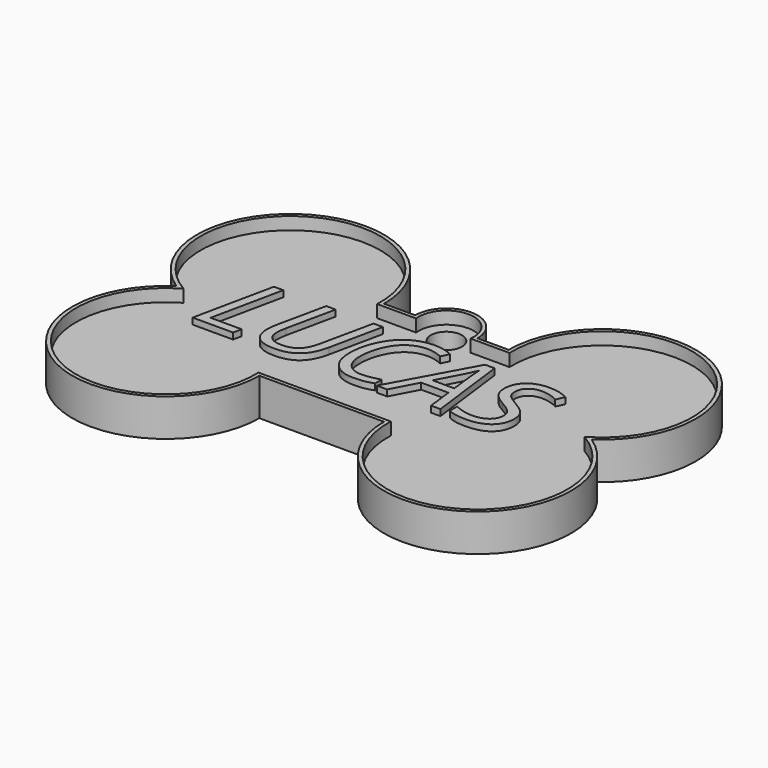
from build123d import *

# Parameters (mm, degrees)
F0_R         = 2.5
F1_DEPTH     = 4
F3_DEPTH     = 2
F4_TEXT_SIZE = 18.0555555556
F5_DEPTH     = 1


# Not quite as in the source:
# - Text() gives the source's letters only with a copy of the font that has no kerning and outlines rounded to 1/6400 em; it was checked with that copy


with BuildPart() as f1:
    # F0 (on Top) → F1 (new body)
    with BuildSketch(Plane.XY):
        with BuildLine():
            Line((-5, 12.5), (-10, 12.5))
            ThreePointArc((-10, 12.5), (-32.0931858273, 25.7169101843), (-33.2915619759, 0))
            ThreePointArc((-33.2915619759, 0), (-32.0931858273, -25.7169101843), (-10, -12.5))
            Line((-10, -12.5), (10, -12.5))
            ThreePointArc((10, -12.5), (32.0931858273, -25.7169101843), (33.2915619759, 0))
            ThreePointArc((33.2915619759, 0), (32.0931858273, 25.7169101843), (10, 12.5))
            Line((10, 12.5), (5, 12.5))
            ThreePointArc((5, 12.5), (0, 17.5), (-5, 12.5))
        make_face()
        with Locations((0, 12.5)):
            Circle(F0_R, mode=Mode.SUBTRACT)
    extrude(amount=F1_DEPTH)

    # F2 (on face) → F3 (join)
    with BuildSketch(Plane.XY.offset(4)):
        with BuildLine():
            ThreePointArc((33.2915619759, 0), (32.0931858273, 25.7169101843), (10, 12.5))
            Line((10, 12.5), (5, 12.5))
            ThreePointArc((5, 12.5), (0, 17.5), (-5, 12.5))
            Line((-5, 12.5), (-10, 12.5))
            ThreePointArc((-10, 12.5), (-32.0931858273, 25.7169101843), (-33.2915619759, 0))
            ThreePointArc((-33.2915619759, 0), (-32.0931858273, -25.7169101843), (-10, -12.5))
            Line((-10, -12.5), (10, -12.5))
            ThreePointArc((10, -12.5), (32.0931858273, -25.7169101843), (33.2915619759, 0))
        make_face()
        with BuildLine():
            ThreePointArc((-10.6125054301, -11.9), (-31.9642656137, -25.1039281362), (-32.1491258207, 0))
            ThreePointArc((-32.1491258207, 0), (-31.9642656137, 25.1039281362), (-10.6125054301, 11.9))
            Line((-10.6125054301, 11.9), (-4.3588989435, 11.9))
            ThreePointArc((-4.3588989435, 11.9), (0, 16.9), (4.3588989435, 11.9))
            Line((4.3588989435, 11.9), (10.6125054301, 11.9))
            ThreePointArc((10.6125054301, 11.9), (31.9642656137, 25.1039281362), (32.1491258207, 0))
            ThreePointArc((32.1491258207, 0), (31.9642656137, -25.1039281362), (10.6125054301, -11.9))
            Line((10.6125054301, -11.9), (-10.6125054301, -11.9))
        make_face(mode=Mode.SUBTRACT)
    extrude(amount=F3_DEPTH)


with BuildPart() as f5:
    # F4 (on face) → F5 (new body)
    with BuildSketch(Plane.XY.offset(6)):
        with Locations((-25.9266493056, -6.9)):
            Text('LUCAS', F4_TEXT_SIZE, font='Open Sans', font_style=FontStyle.ITALIC, text_align=(TextAlign.LEFT, TextAlign.BOTTOM))
    extrude(amount=F5_DEPTH)


solid = Compound([f1.part, f5.part])
